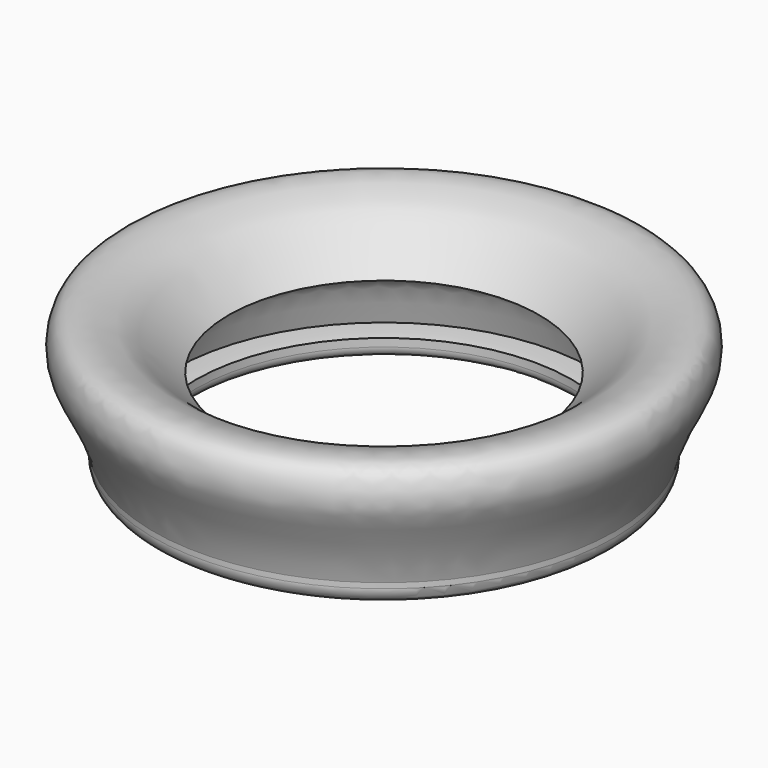
from build123d import *

# Parameters (mm, degrees)
F3_R = 0.5
F4_R = 0.75


with BuildPart() as f1:
    # F0 (on Front) → F1 (revolve)
    with BuildSketch(Plane.XZ):
        with BuildLine():
            add(Edge.make_bspline(
                [(-9.9, 2), (-9.5758501784, 2), (-9.2390440685, 1.9540368163), (-8.9, 1.8756836241)],
                knots=[0, 0, 0, 0, 0.9057827175, 0.9057827175, 0.9057827175, 0.9057827175], degree=3))
            add(Edge.make_bspline(
                [(-9.9, 2), (-9.4425315337, 3.4727421793), (-9.475417137, 4.1546168904), (-7.8504308779, 4.8879319086), (-7.3364856621, 5.0781547656)],
                knots=[0, 0, 0, 0, 0.3609898147, 0.4924868102, 0.4924868102, 0.4924868102, 0.4924868102], degree=3))
            add(Edge.make_bspline(
                [(-7.3364856621, 5.0781547656), (-7.8661996988, 5.5186899413), (-8.9848796151, 6.6731469392), (-10.2827477013, 7.4070818452), (-12.2553368007, 7.6610451612), (-12.6137007512, 5.9133238981), (-11.9614741658, 4.6431108193), (-11.1182323438, 3.0212863117), (-10.9, 2)],
                knots=[0, 0, 0, 0, 0.1855602792, 0.3413856413, 0.4983155684, 0.6419424505, 0.7899465755, 1, 1, 1, 1], degree=3))
            Line((-10.9, 2), (-10.9, 1))
            Line((-10.9, 1), (-8.9, 1))
            Line((-8.9, 1), (-8.9, 1.8756836241))
        make_face()
    revolve(axis=Axis((0, 0, 3.25), (0, 0, 1)))

    # F3
    f3_edges = [f1.edges().sort_by_distance(p)[0] for p in [
        (8.9, 0, 1),
    ]]
    fillet(f3_edges, radius=F3_R)

    # F4
    f4_edges = [f1.edges().sort_by_distance(p)[0] for p in [
        (10.9, 0, 1),
    ]]
    fillet(f4_edges, radius=F4_R)


solid = f1.part
